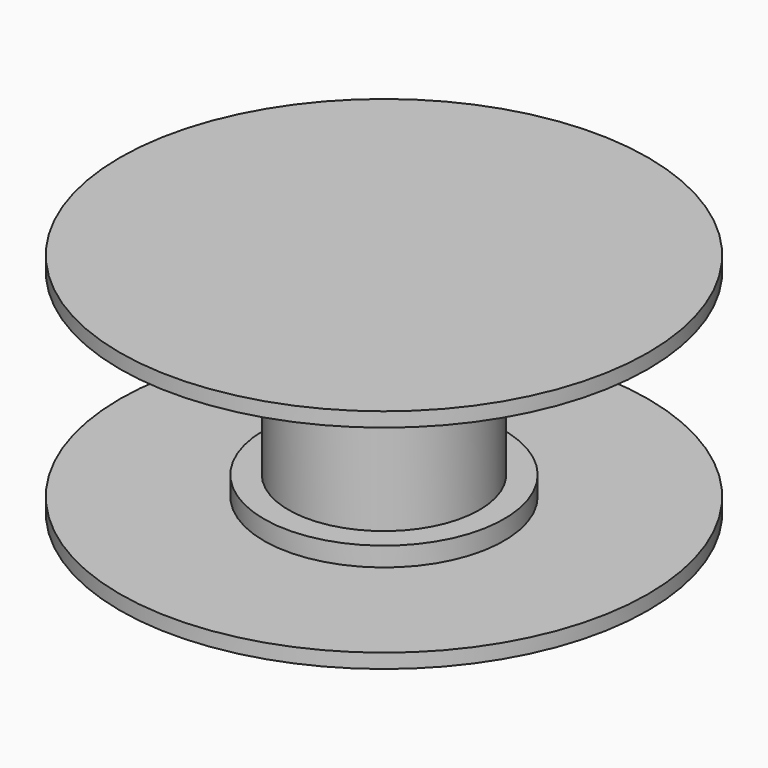
from build123d import *

# Parameters (mm, degrees)
F0_W     = 5
F0_H     = 0.8
F2_R     = 3.975
F2_R_2   = 2.975
F3_DEPTH = 6.65
F5_R     = 2.975
F6_DEPTH = 6


# Not quite as in the source:
# - a feature names something its author has since deleted; it is built from what else it names


with BuildPart() as f1:
    # F0 (on Front) → F1 (revolve)
    with BuildSketch(Plane.XZ):
        with Locations((-2.5, 0.4)):
            Rectangle(F0_W, F0_H)
        Polygon((0, -0.6), (0, 0), (-5, 0), (-11, 0), (-11, -0.6), (-10.4, -0.6), align=None)
    revolve(axis=Axis((0, 0, 3.9109135978), (0, 0, -1)))

    # F2 (on face) → F3 (join)
    with BuildSketch(Plane.XY.offset(0.8)):
        Circle(F2_R)
        Circle(F2_R_2, mode=Mode.SUBTRACT)
    extrude(amount=F3_DEPTH)


with BuildPart() as f4:
    # F0 (on Front) → F4 (revolve)
    with BuildSketch(Plane.XZ):
        Polygon((-11, 8.85), (-11, 8.25), (-5, 8.25), (0, 8.25), (0, 8.85), (-10.4, 8.85), align=None)
        with Locations((-2.5, 7.85)):
            Rectangle(F0_W, F0_H)
    revolve(axis=Axis((0, 0, 3.9109135978), (0, 0, -1)))

    # F5 (on face) → F6 (join)
    with BuildSketch(Plane(origin=(0, 0, 7.45), x_dir=(1, 0, 0), z_dir=(0, 0, -1))):
        Circle(F5_R)
    extrude(amount=F6_DEPTH)


solid = Compound([f1.part, f4.part])
